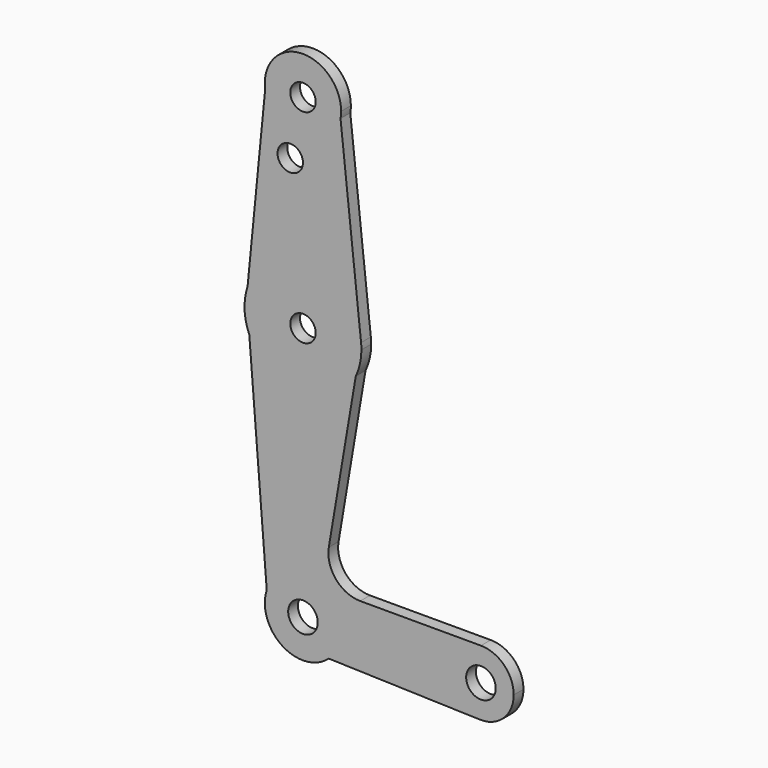
from build123d import *

# Parameters (mm, degrees)
F0_R     = 3.175
F0_R_2   = 3.6935498759
F1_DEPTH = 3.048


# Not quite as in the source:
# - the program builds the solid bodies; features that only make, move or delete a surface that nothing else refers to are left out


with BuildPart() as f1:
    # F0 (on Front) → F1 (new body)
    with BuildSketch(Plane.XZ):
        with BuildLine():
            ThreePointArc((9.3833145649, 112.6632248852), (9.4895125331, 113.4785519586), (9.525, 114.3))
            ThreePointArc((9.525, 114.3), (-0.6480489734, 123.8029288921), (-9.4368178537, 113.0069053411))
            ThreePointArc((-9.4368178537, 113.0069053411), (-0.1739100757, 104.7765877814), (9.3833145649, 112.6632248852))
        make_face()
        with Locations((0, 114.3)):
            Circle(F0_R, mode=Mode.SUBTRACT)
        with BuildLine():
            ThreePointArc((9.3833145649, 112.6632248852), (-0.1739100757, 104.7765877814), (-9.4368178537, 113.0069053411))
            Line((-9.4368178537, 113.0069053411), (-13.8405466215, 68.1295922048))
            ThreePointArc((-13.8405466215, 68.1295922048), (1.5694846966, 78.00967169), (14.510379821, 65.0629242514))
            Line((14.510379821, 65.0629242514), (9.3833145649, 112.6632248852))
        make_face()
        with Locations((-3.175, 99.886942851)):
            Circle(F0_R, mode=Mode.SUBTRACT)
        with BuildLine():
            ThreePointArc((14.510379821, 65.0629242514), (1.5694846966, 78.00967169), (-13.8405466215, 68.1295922048))
            ThreePointArc((-13.8405466215, 68.1295922048), (-14.0055954943, 67.6033095928), (-14.1506404779, 67.0711663123))
            Line((-14.1506404779, 67.0711663123), (-13.406906479, 57.7338302637))
            ThreePointArc((-13.406906479, 57.7338302637), (-0.26538464, 48.9081041068), (13.1883694151, 57.2501386467))
            Line((13.1883694151, 57.2501386467), (14.510379821, 65.0629242514))
        make_face()
        with Locations((0, 63.5)):
            Circle(F0_R, mode=Mode.SUBTRACT)
        with BuildLine():
            ThreePointArc((14.5943089855, 63.5), (14.5733115895, 64.2825880654), (14.510379821, 65.0629242514))
            Line((14.510379821, 65.0629242514), (13.1883694151, 57.2501386467))
            ThreePointArc((13.1883694151, 57.2501386467), (14.2384864544, 60.2969767012), (14.5943089855, 63.5))
        make_face()
        with BuildLine():
            Line((-13.406906479, 57.7338302637), (-14.1506404779, 67.0711663123))
            ThreePointArc((-14.1506404779, 67.0711663123), (-14.5482321844, 62.3412096509), (-13.406906479, 57.7338302637))
        make_face()
        with BuildLine():
            Line((6.4543763873, 17.4537470642), (13.1883694151, 57.2501386467))
            ThreePointArc((13.1883694151, 57.2501386467), (-0.26538464, 48.9081041068), (-13.406906479, 57.7338302637))
            Line((-13.406906479, 57.7338302637), (-9.0459006939, 2.9828351674))
            ThreePointArc((-9.0459006939, 2.9828351674), (1.5105331659, 9.4044624809), (9.525, 0))
            ThreePointArc((9.525, 0), (8.7148100466, -3.8441788267), (6.4220685875, -7.0343912357))
            Line((6.4220685875, -7.0343912357), (44.2035880522, -8.173426155))
            ThreePointArc((44.2035880522, -8.173426155), (36.2737887259, 0.1232199644), (44.45, 8.1771397175))
            Line((44.45, 8.1771397175), (14.2931469281, 8.1771397175))
            ThreePointArc((14.2931469281, 8.1771397175), (8.220631645, 10.996039865), (6.4543763873, 17.4537470642))
        make_face()
        with BuildLine():
            ThreePointArc((9.525, 0), (1.5105331659, 9.4044624809), (-9.0459006939, 2.9828351674))
            ThreePointArc((-9.0459006939, 2.9828351674), (-5.1775795439, -7.9948918108), (6.4220685875, -7.0343912357))
            ThreePointArc((6.4220685875, -7.0343912357), (8.7148100466, -3.8441788267), (9.525, 0))
        make_face()
        Circle(F0_R_2, mode=Mode.SUBTRACT)
        with BuildLine():
            ThreePointArc((52.6271397175, 0), (50.2321109449, 5.7821109449), (44.45, 8.1771397175))
            ThreePointArc((44.45, 8.1771397175), (36.2737887259, 0.1232199644), (44.2035880522, -8.173426155))
            ThreePointArc((44.2035880522, -8.173426155), (50.1443247639, -5.8685841088), (52.6271397175, 0))
        make_face()
        with Locations((44.45, 0)):
            Circle(F0_R_2, mode=Mode.SUBTRACT)
    extrude(amount=F1_DEPTH)


solid = f1.part
